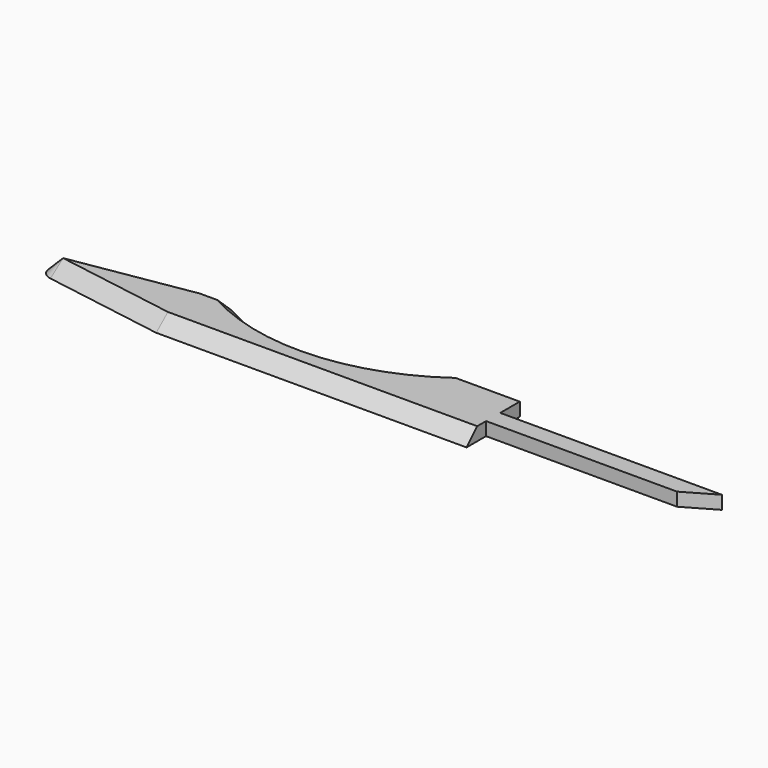
from build123d import *

# Parameters (mm, degrees)
F1_DEPTH = 3
F2_SIZE  = 2.99999


# Not quite as in the source:
# - a fillet or chamfer is up to 0.001 mm smaller than in the source, because OpenCascade refuses the exact size


with BuildPart() as f1:
    # F0 (on Top) → F1 (new body)
    with BuildSketch(Plane.XY):
        with BuildLine():
            Line((0, 2), (0, 7.5))
            Line((0, 7.5), (-20, 7.5))
            ThreePointArc((-20, 7.5), (-42.5, 1.4711431703), (-65, 7.5))
            Line((-65, 7.5), (-70, 7.5))
            Line((-70, 7.5), (-70, 0))
            Line((-70, 0), (-70, -7.5))
            Line((-70, -7.5), (0, -7.5))
            Line((0, -7.5), (0, -2))
            Line((0, -2), (0, 0))
            Line((0, 0), (0, 2))
        make_face()
        Polygon((50, 2), (0, 2), (0, 0), (0, -2), (43.0717967697, -2), align=None)
        with BuildLine():
            Line((-70, 0), (-70, 7.5))
            Line((-70, 7.5), (-97.4888614164, 2.959901099))
            ThreePointArc((-97.4888614164, 2.959901099), (-99.2876389848, 1.9408008335), (-100, 0))
            Line((-100, 0), (-70, 0))
        make_face()
        with BuildLine():
            Line((-70, -7.5), (-70, 0))
            Line((-70, 0), (-100, 0))
            ThreePointArc((-100, 0), (-99.2876389848, -1.9408008335), (-97.4888614164, -2.959901099))
            Line((-97.4888614164, -2.959901099), (-70, -7.5))
        make_face()
    extrude(amount=F1_DEPTH)

    # F2 (size 3 in the source; OpenCascade refuses exactly that, so slightly less here)
    f2_edges = [f1.edges().sort_by_distance(p)[0] for p in [
        (-42.5, 1.471143, 3),
        (-83.744431, 5.229951, 3),
        (-67.5, 7.5, 3),
        (-100, 0, 3),
        (-83.744431, -5.229951, 3),
        (-35, -7.5, 3),
    ]]
    chamfer(f2_edges, length=F2_SIZE)


solid = f1.part
